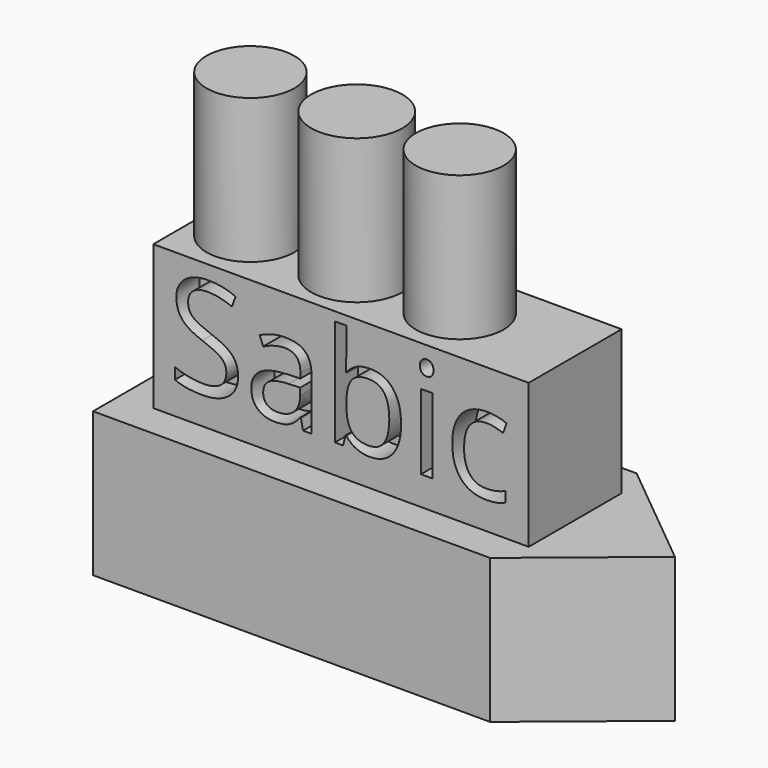
from build123d import *

# Parameters (mm, degrees)
F1_DEPTH      = 25.4
F2_W          = 66.04
F2_H          = 20.4370947814
F3_DEPTH      = 50.8
F4_R          = 7.7293397339
F6_DEPTH      = 76.2
F5_R          = 8.0328555842
F7_DEPTH      = 76.2
F8_R          = 7.7279041071
F9_DEPTH      = 76.2
F10_TEXT_SIZE = 24.6944444444
F11_DEPTH     = 5.08


# Not quite as in the source:
# - Text() gives the source's letters only with a copy of the font that has no kerning and outlines rounded to 1/6400 em; it was checked with that copy


with BuildPart() as f1:
    # F0 (on Top) → F1 (new body)
    with BuildSketch(Plane.XY):
        Polygon((11.1665374938, 16.1127906742), (-58.6834625062, 16.1127906742), (-58.6834625062, -16.1127906742), (11.1665374938, -16.1127906742), (30.8016584939, 0), align=None)
    extrude(amount=F1_DEPTH)

    # F2 (on Top) → F3 (join)
    with BuildSketch(Plane.XY):
        with Locations((-19.7706625062, -0.0014432835)):
            Rectangle(F2_W, F2_H)
    extrude(amount=F3_DEPTH)

    # F4 (on Top) → F6 (join)
    with BuildSketch(Plane.XY):
        with Locations((-43.8903793693, 0)):
            Circle(F4_R)
    extrude(amount=F6_DEPTH)

    # F5 (on Top) → F7 (join)
    with BuildSketch(Plane.XY):
        with Locations((-25.1830033958, 0)):
            Circle(F5_R)
    extrude(amount=F7_DEPTH)

    # F8 (on Top) → F9 (join)
    with BuildSketch(Plane.XY):
        with Locations((-7.0698018475, 0)):
            Circle(F8_R)
    extrude(amount=F9_DEPTH)

    # F10 (on face) → F11 (cut)
    with BuildSketch(Plane.XZ.offset(10.2199906742)):
        with Locations((-50.2506625062, 30.48)):
            Text('Sabic', F10_TEXT_SIZE, font='Open Sans', text_align=(TextAlign.LEFT, TextAlign.BOTTOM))
    extrude(amount=-F11_DEPTH, mode=Mode.SUBTRACT)


solid = f1.part
